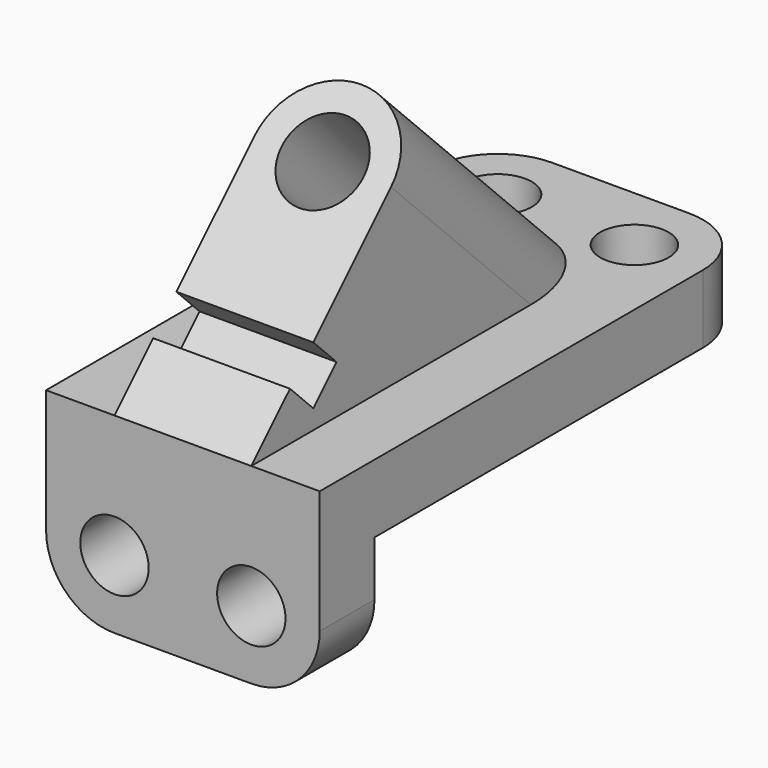
from build123d import *

# Parameters (mm, degrees)
F0_W           = 100
F0_H           = 70
F1_DEPTH       = 200
F2_R           = 25
F3_T           = -25
F5_START       = -25
F5_DEPTH       = 50
F6_R           = 24.99999
F9_D           = 25
F9_DEPTH       = 100
F9_TIP         = 7.5107577378
F9_ON_F8_D     = 25
F9_ON_F8_DEPTH = 100
F9_ON_F8_TIP   = 7.5107577378
F10_R          = 15
F11_DEPTH      = 50


# Not quite as in the source:
# - a fillet or chamfer is up to 0.001 mm smaller than in the source, because OpenCascade refuses the exact size


with BuildPart() as f1:
    # F0 (on Front) → F1 (new body)
    with BuildSketch(Plane.XZ):
        with Locations((50, -35)):
            Rectangle(F0_W, F0_H)
    extrude(amount=-F1_DEPTH)

    # F2
    f2_edges = [f1.edges().sort_by_distance(p)[0] for p in [
        (100, 100, -70),
        (0, 100, -70),
        (100, 200, -35),
        (0, 200, -35),
    ]]
    fillet(f2_edges, radius=F2_R)

    # F3
    f3_openings = [f1.faces().sort_by_distance(p)[0] for p in [
        (100, 87.5, -22.5),
        (50, 200, -35),
        (92.67767, 192.67767, -35),
        (7.32233, 192.67767, -35),
        (0, 87.5, -22.5),
        (92.67767, 100, -62.67767),
        (50, 100, -70),
        (7.32233, 100, -62.67767),
    ]]
    offset(amount=F3_T, openings=f3_openings)

    # F4 (on face) → F5 (join)
    with BuildSketch(Plane.YZ.offset(100).offset(F5_START)):
        Polygon((17.6776695297, 17.6776695297), (0, 0), (163, 0), (81.5, 81.5), (28.2842712475, 28.2842712475), (38.8908729653, 17.6776695297), (28.2842712475, 7.0710678119), align=None)
    extrude(amount=-F5_DEPTH)

    # F6 (radius 25 in the source; OpenCascade refuses exactly that, so slightly less here)
    f6_edges = [f1.edges().sort_by_distance(p)[0] for p in [
        (75, 122.25, 40.75),
        (25, 122.25, 40.75),
    ]]
    fillet(f6_edges, radius=F6_R)

    # F9
    with Locations(Plane.XZ):
        with Locations((75, -45), (25, -45)):
            Hole(F9_D / 2, depth=F9_DEPTH)
            with Locations((0, 0, -(F9_DEPTH + F9_TIP / 2))):  # 118° drill point
                Cone(0, F9_D / 2, F9_TIP, mode=Mode.SUBTRACT)

    # F9 on F8
    with Locations(Plane.XY):
        with Locations((75, 175), (25, 175)):
            Hole(F9_ON_F8_D / 2, depth=F9_ON_F8_DEPTH)
            with Locations((0, 0, -(F9_ON_F8_DEPTH + F9_ON_F8_TIP / 2))):  # 118° drill point
                Cone(0, F9_ON_F8_D / 2, F9_ON_F8_TIP, mode=Mode.SUBTRACT)

    # F10 (on face) → F11 (cut)
    with BuildSketch(Plane(origin=(0, 0, 0), x_dir=(1, 0, 0), z_dir=(0, -0.7071067812, 0.7071067812))):
        with Locations((50, 90.2584053334)):
            Circle(F10_R)
    extrude(amount=-F11_DEPTH, mode=Mode.SUBTRACT)


solid = f1.part
